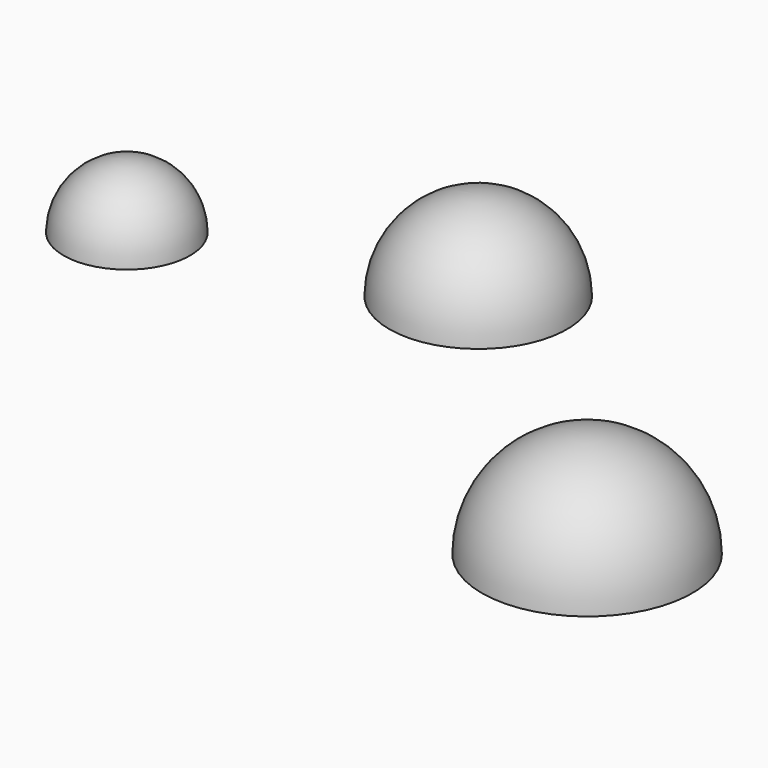
from build123d import *

# Parameters (mm, degrees)
F6_S5_R       = 5.2
F6_T6_DEPTH   = 9
F6_2_S5_R     = 5.2
F6_2_T6_DEPTH = 9
F6_3_S5_R     = 4.2
F6_3_T6_DEPTH = 8


# Not quite as in the source:
# - a fillet or chamfer that OpenCascade refuses, or shapes differently, is made with other operations: its cross-section is extruded or revolved along the edge and cut away or added


with BuildPart() as f1:
    # F0 (on Front) → F1 (revolve)
    with BuildSketch(Plane.XZ):
        with BuildLine():
            Line((-85.4260504544, 34.7033580244), (-85.4260504544, 35.7033580244))
            ThreePointArc((-85.4260504544, 35.7033580244), (-94.9719920004, 31.7492995704), (-98.9260504544, 22.2033580244))
            Line((-98.9260504544, 22.2033580244), (-90.6260504544, 22.2033580244))
            Line((-90.6260504544, 22.2033580244), (-90.6260504544, 27.4033580244))
            Line((-90.6260504544, 27.4033580244), (-87.6760504544, 27.4033580244))
            Line((-87.6760504544, 27.4033580244), (-87.6760504544, 34.7033580244))
            Line((-87.6760504544, 34.7033580244), (-85.4260504544, 34.7033580244))
        make_face()
    revolve(axis=Axis((-85.4260504544, 0, 28.9533580244), (0, 0, 1)))

    # F6: chamfer of 3 on 1 edges, made by hand


with BuildPart() as f3:
    # F2 (on Front) → F3 (revolve)
    with BuildSketch(Plane.XZ):
        with BuildLine():
            Line((12.9549296586, 15.1117370081), (12.9549296586, 16.1117370081))
            ThreePointArc((12.9549296586, 16.1117370081), (-2.9549729181, 9.5216395848), (-9.5450703414, -6.3882629919))
            Line((-9.5450703414, -6.3882629919), (7.7549296586, -6.3882629919))
            Line((7.7549296586, -6.3882629919), (7.7549296586, -1.1882629919))
            Line((7.7549296586, -1.1882629919), (10.7049296586, -1.1882629919))
            Line((10.7049296586, -1.1882629919), (10.7049296586, 15.1117370081))
            Line((10.7049296586, 15.1117370081), (12.9549296586, 15.1117370081))
        make_face()
    revolve(axis=Axis((12.9549296586, 0, 4.8617370081), (0, 0, 1)))

    # F6#2: chamfer of 3 on 1 edges, made by hand


with BuildPart() as f5:
    # F4 (on Front) → F5 (revolve)
    with BuildSketch(Plane.XZ):
        with BuildLine():
            Line((-10.3169069651, 52.5661451879), (-10.3169069651, 53.5661451879))
            ThreePointArc((-10.3169069651, 53.5661451879), (-23.7519358077, 48.0011740305), (-29.3169069651, 34.5661451879))
            Line((-29.3169069651, 34.5661451879), (-14.5169069651, 34.5661451879))
            Line((-14.5169069651, 34.5661451879), (-14.5169069651, 38.5661451879))
            Line((-14.5169069651, 38.5661451879), (-12.0669069651, 38.5661451879))
            Line((-12.0669069651, 38.5661451879), (-12.0669069651, 52.5661451879))
            Line((-12.0669069651, 52.5661451879), (-10.3169069651, 52.5661451879))
        make_face()
    revolve(axis=Axis((-10.3169069651, 0, 44.0661451879), (0, 0, 1)))

    # F6#3: chamfer of 3 on 1 edges, made by hand


with BuildPart() as f6_tool2:
    # F6_s3 → F6_t4 (revolve)
    with BuildSketch(Plane.XZ):
        Polygon((-90.6760504544, 27.4033580244), (-87.6760504544, 30.4033580244), (-87.6760504544, 27.4033580244), align=None)
    revolve(axis=Axis((-85.4260504544, 0, 27.4033580244), (0, 0, 1)))

    # F6_s5 → F6_t6 (intersect, symmetric)
    with BuildSketch(Plane.XY.offset(28.9)):
        with Locations((-85.4260504544, 0)):
            Circle(F6_S5_R)
    extrude(amount=F6_T6_DEPTH, both=True, mode=Mode.INTERSECT)


with BuildPart() as f1_1:
    add(f1.part)

    # F6_t1: cut F6_tool2
    add(f6_tool2.part, mode=Mode.SUBTRACT)

    # F7: chamfer of 1 on 1 edges, made by hand

    # F7_s1 → F7_t2 (revolve, cut)
    with BuildSketch(Plane.XZ):
        Polygon((-91.6260504544, 22.2033580244), (-90.6260504544, 23.2033580244), (-90.6260504544, 22.2033580244), align=None)
    revolve(axis=Axis((-85.4260504544, 0, 22.2033580244), (0, 0, 1)), mode=Mode.SUBTRACT)


with BuildPart() as f6_2_tool2:
    # F6_2_s3 → F6_2_t4 (revolve)
    with BuildSketch(Plane.XZ):
        Polygon((10.7049296586, 1.8117370081), (7.7049296586, -1.1882629919), (10.7049296586, -1.1882629919), align=None)
    revolve(axis=Axis((12.9549296586, 0, -1.1882629919), (0, 0, 1)))

    # F6_2_s5 → F6_2_t6 (intersect, symmetric)
    with BuildSketch(Plane.XY.offset(0.3)):
        with Locations((12.9549296586, 0)):
            Circle(F6_2_S5_R)
    extrude(amount=F6_2_T6_DEPTH, both=True, mode=Mode.INTERSECT)


with BuildPart() as f3_1:
    add(f3.part)

    # F6_2_t1: cut F6_2_tool2
    add(f6_2_tool2.part, mode=Mode.SUBTRACT)

    # F7#3: chamfer of 1 on 1 edges, made by hand

    # F7_3_s1 → F7_3_t2 (revolve, cut)
    with BuildSketch(Plane.XZ):
        Polygon((7.7549296586, -5.3882629919), (6.7549296586, -6.3882629919), (7.7549296586, -6.3882629919), align=None)
    revolve(axis=Axis((12.9549296586, 0, -6.3882629919), (0, 0, 1)), mode=Mode.SUBTRACT)


with BuildPart() as f6_3_tool2:
    # F6_3_s3 → F6_3_t4 (revolve)
    with BuildSketch(Plane.XZ):
        Polygon((-15.0669069651, 38.5661451879), (-12.0669069651, 41.5661451879), (-12.0669069651, 38.5661451879), align=None)
    revolve(axis=Axis((-10.3169069651, 0, 38.5661451879), (0, 0, 1)))

    # F6_3_s5 → F6_3_t6 (intersect, symmetric)
    with BuildSketch(Plane.XY.offset(40.1)):
        with Locations((-10.3169069651, 0)):
            Circle(F6_3_S5_R)
    extrude(amount=F6_3_T6_DEPTH, both=True, mode=Mode.INTERSECT)


with BuildPart() as f5_1:
    add(f5.part)

    # F6_3_t1: cut F6_3_tool2
    add(f6_3_tool2.part, mode=Mode.SUBTRACT)

    # F7#2: chamfer of 1 on 1 edges, made by hand

    # F7_2_s1 → F7_2_t2 (revolve, cut)
    with BuildSketch(Plane.XZ):
        Polygon((-15.5169069651, 34.5661451879), (-14.5169069651, 35.5661451879), (-14.5169069651, 34.5661451879), align=None)
    revolve(axis=Axis((-10.3169069651, 0, 34.5661451879), (0, 0, 1)), mode=Mode.SUBTRACT)


solid = Compound([f1_1.part, f3_1.part, f5_1.part])
